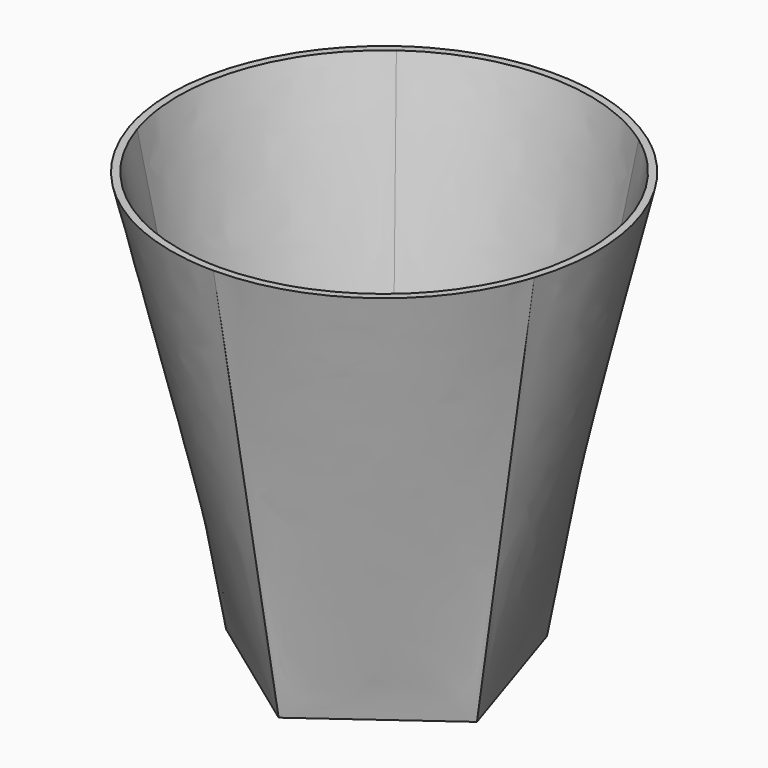
from build123d import *

# Parameters (mm, degrees)
F4_T = 1.27


# Not quite as in the source:
# - the arcs of a loft's sections are written as splines that run evenly, so that the points pair up as in the source's solid
# - a shell that OpenCascade refuses in one call is made with other operations: the cavity is built on its own and cut out


with BuildPart() as f3:
    # F2 (on offset) → F3 section 0
    with BuildSketch(Plane.XY.offset(76.2)):
        with BuildLine():
            add(Edge.make_bspline(
                [(22.3946181123, 30.8235474857), (19.1667837677, 33.1687064104), (15.5680943349, 35.0023302613), (7.9790006365, 37.4681762804), (3.9898226701, 38.1), (-3.9898226701, 38.1), (-7.9790006365, 37.4681762804), (-15.5680943349, 35.0023302613), (-19.1667837677, 33.1687064104), (-22.3946181123, 30.8235474857)],
                knots=[0, 0, 0, 0, 0.25, 0.25, 0.5, 0.5, 0.75, 0.75, 1, 1, 1, 1], degree=3))
            add(Edge.make_bspline(
                [(-22.3946181123, 30.8235474857), (-25.622452457, 28.478388561), (-28.478388561, 25.622452457), (-33.1687064104, 19.1667837677), (-35.0023302613, 15.5680943349), (-37.4681762804, 7.9790006365), (-38.1, 3.9898226701), (-38.1, -3.9898226701), (-37.4681762804, -7.9790006365), (-36.2352532708, -11.7735474857)],
                knots=[0, 0, 0, 0, 0.25, 0.25, 0.5, 0.5, 0.75, 0.75, 1, 1, 1, 1], degree=3))
            add(Edge.make_bspline(
                [(-36.2352532708, -11.7735474857), (-35.0023302613, -15.5680943349), (-33.1687064104, -19.1667837677), (-28.478388561, -25.622452457), (-25.622452457, -28.478388561), (-19.1667837677, -33.1687064104), (-15.5680943349, -35.0023302613), (-7.9790006365, -37.4681762804), (-3.9898226701, -38.1), (0, -38.1)],
                knots=[0, 0, 0, 0, 0.25, 0.25, 0.5, 0.5, 0.75, 0.75, 1, 1, 1, 1], degree=3))
            add(Edge.make_bspline(
                [(0, -38.1), (3.9898226701, -38.1), (7.9790006365, -37.4681762804), (15.5680943349, -35.0023302613), (19.1667837677, -33.1687064104), (25.622452457, -28.478388561), (28.478388561, -25.622452457), (33.1687064104, -19.1667837677), (35.0023302613, -15.5680943349), (36.2352532708, -11.7735474857)],
                knots=[0, 0, 0, 0, 0.25, 0.25, 0.5, 0.5, 0.75, 0.75, 1, 1, 1, 1], degree=3))
            add(Edge.make_bspline(
                [(36.2352532708, -11.7735474857), (37.4681762804, -7.9790006365), (38.1, -3.9898226701), (38.1, 3.9898226701), (37.4681762804, 7.9790006365), (35.0023302613, 15.5680943349), (33.1687064104, 19.1667837677), (28.478388561, 25.622452457), (25.622452457, 28.478388561), (22.3946181123, 30.8235474857)],
                knots=[0, 0, 0, 0, 0.25, 0.25, 0.5, 0.5, 0.75, 0.75, 1, 1, 1, 1], degree=3))
        make_face()
    # F0 (on Top) → F3 section 1
    with BuildSketch(Plane.XY):
        Polygon((13.8406351585, 19.05), (-13.8406351585, 19.05), (-22.3946181123, -7.2764525143), (0, -23.5470949714), (22.3946181123, -7.2764525143), align=None)
    loft(ruled=True)

    # F4: shell of thickness 1.27, made by hand


with BuildPart() as f4_core1:
    # F4_t2: copy of F3
    add(f3.part)

    # the walls: a layer under each face that stays
    f4_faces = [f4_core1.faces().sort_by_distance(p)[0] for p in [
        (0, 28.575, 38.1),
        (-27.1764399531, 8.8301606143, 38.1),
        (-16.7959635843, -23.1176606143, 38.1),
        (16.7959635843, -23.1176606143, 38.1),
        (27.1764399531, 8.8301606143, 38.1),
        (-1.3216630512, 1.8191131286, 0),
    ]]
    thicken(f4_faces, amount=-F4_T, mode=Mode.SUBTRACT)


with BuildPart() as f3_1:
    add(f3.part)

    # what is left inside the walls is the cavity
    f4_cavity = [f4_core1.part.solids().sort_by_distance(p)[0] for p in [
        (10.168811, -6.868871, 76.1873),
    ]]
    add(f4_cavity, mode=Mode.SUBTRACT)


solid = f3_1.part
